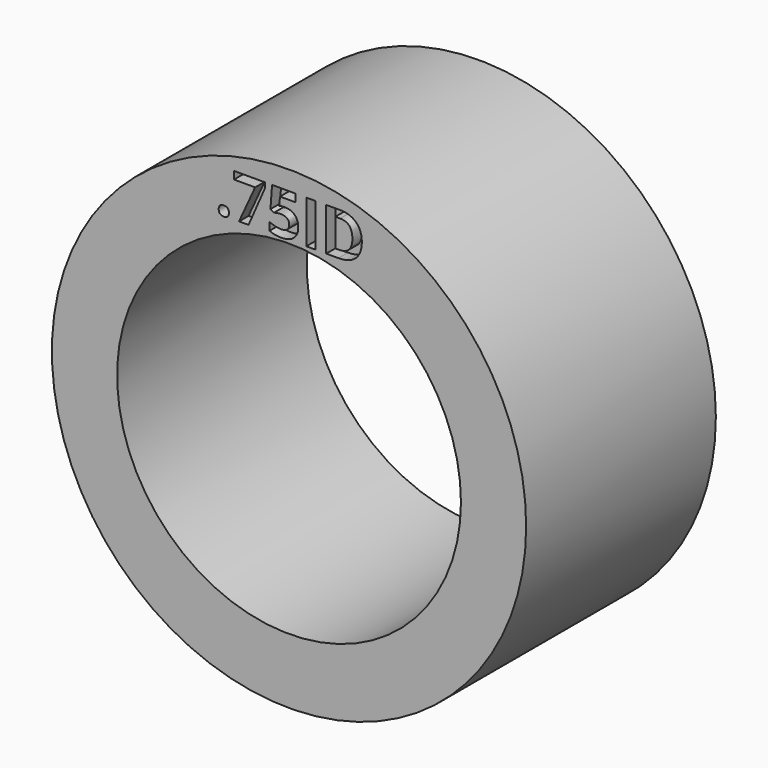
from build123d import *

# Parameters (mm, degrees)
F0_R         = 12.7
F0_R_2       = 9.2075
F1_DEPTH     = 12.7
F2_TEXT_SIZE = 3.2170675695
F3_DEPTH     = 0.635


# Not quite as in the source:
# - Text() gives the source's letters only with a copy of the font that has no kerning and outlines rounded to 1/6400 em; it was checked with that copy


with BuildPart() as f1:
    # F0 (on Front) → F1 (new body)
    with BuildSketch(Plane.XZ):
        Circle(F0_R)
        Circle(F0_R_2, mode=Mode.SUBTRACT)
    extrude(amount=-F1_DEPTH)

    # F2 (on face) → F3 (cut)
    with BuildSketch(Plane.XZ):
        with Locations((-3.9511267096, 9.375798516)):
            Text('.75ID', F2_TEXT_SIZE, font='Open Sans', font_style=FontStyle.BOLD, text_align=(TextAlign.LEFT, TextAlign.BOTTOM))
    extrude(amount=-F3_DEPTH, mode=Mode.SUBTRACT)


solid = f1.part
